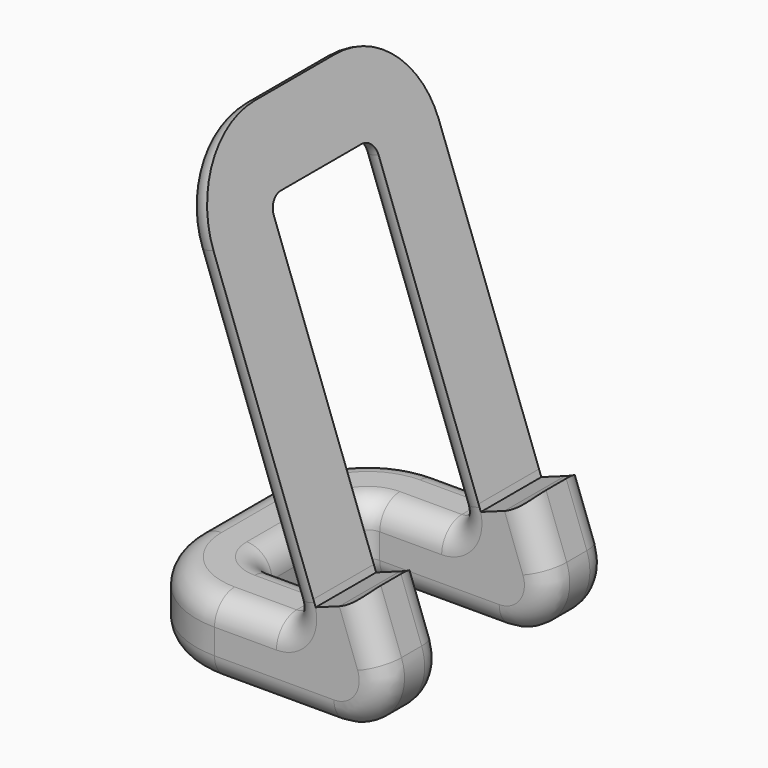
from build123d import *

# Parameters (mm, degrees)
F1_DEPTH     = 56
F2_W         = 41
F2_H         = 26
F3_DEPTH     = 15
F4_W         = 26
F4_H         = 80
F5_DEPTH     = 15
F6_R         = 10
F7_R         = 18
F8_R         = 3
F9_T1_DEPTH  = 58.556339633
F9_T3_DEPTH  = 12.2933358786
F9_T5_DEPTH  = 23.7185199326
F9_T7_DEPTH  = 24.4815236869
F9_T9_DEPTH  = 20
F9_T11_DEPTH = 58.556339633
F9_T13_DEPTH = 24.4815236869
F9_T16_ANGLE = 90
F9_T18_ANGLE = 110
F9_T20_ANGLE = 110
F9_T22_ANGLE = 110
F9_T24_ANGLE = 90
F9_T26_ANGLE = 90
F9_T28_ANGLE = 90
F9_T30_ANGLE = 90
F9_T32_ANGLE = 110
F9_T34_ANGLE = 90
F9_T36_ANGLE = 90
F9_T38_ANGLE = 90
F9_T40_ANGLE = 90
F9_T42_ANGLE = 90
F9_T44_ANGLE = 90
F9_T46_ANGLE = 90
F9_T48_ANGLE = 110
F9_T50_ANGLE = 110
F9_T52_ANGLE = 110
F9_T54_ANGLE = 110


# Not quite as in the source:
# - a fillet or chamfer that OpenCascade refuses, or shapes differently, is made with other operations: its cross-section is extruded or revolved along the edge and cut away or added


with BuildPart() as f1:
    # F0 (on Front) → F1 (new body)
    with BuildSketch(Plane.XZ):
        with BuildLine():
            Line((37.6205974839, 21.2589493944), (11.6270665912, 92.6755885741))
            Line((11.6270665912, 92.6755885741), (6.9286034872, 90.9654878575))
            Line((6.9286034872, 90.9654878575), (34.5777798989, 15))
            Line((34.5777798989, 15), (0, 15))
            Line((0, 15), (0, 0))
            Line((0, 0), (56, 0))
            Line((56, 0), (47.0175236918, 24.6791508276))
            ThreePointArc((47.0175236918, 24.6791508276), (45.0928436241, 22.9155064816), (42.7772806938, 21.7101007166))
            Line((42.7772806938, 21.7101007166), (38.0788175899, 20))
            Line((38.0788175899, 20), (37.6205974839, 21.2589493944))
        make_face()
    extrude(amount=F1_DEPTH)

    # F2 (on face) → F3 (cut, through all)
    with BuildSketch(Plane(origin=(0, 0, 0), x_dir=(1, 0, 0), z_dir=(0, 0, -1))):
        with Locations((35.5, 28)):
            Rectangle(F2_W, F2_H)
    extrude(amount=-F3_DEPTH, mode=Mode.SUBTRACT)

    # F4 (on face) → F5 (cut, through all)
    with BuildSketch(Plane(origin=(35.3538550955, 0, 12.8677509213), x_dir=(0, -1, 0), z_dir=(-0.9396926208, 0, -0.3420201433))):
        with Locations((28, 28.1098757281)):
            Rectangle(F4_W, F4_H)
    extrude(amount=-F5_DEPTH, mode=Mode.SUBTRACT)

    # F6
    f6_edges = [f1.edges().sort_by_distance(p)[0] for p in [
        (56, -7.5, 0),
        (56, -48.5, 0),
    ]]
    fillet(f6_edges, radius=F6_R)

    # F7
    f7_edges = [f1.edges().sort_by_distance(p)[0] for p in [
        (0, -56, 7.5),
        (0, 0, 7.5),
        (9.277835, -56, 91.820538),
        (9.277835, 0, 91.820538),
    ]]
    fillet(f7_edges, radius=F7_R)

    # F8
    f8_edges = [f1.edges().sort_by_distance(p)[0] for p in [
        (15, -15, 7.5),
        (15, -41, 7.5),
        (14.408137, -15, 77.725149),
        (14.408137, -41, 77.725149),
        (34.57778, -7.5, 15),
        (34.57778, -48.5, 15),
    ]]
    fillet(f8_edges, radius=F8_R)

    # F9: fillet of radius 5 on 42 edges, made by hand

    # F9_s2 → F9_t1 (cut)
    with BuildSketch(Plane(origin=(-22.2688890284, 0, 61.183269762), x_dir=(0, 1, 0), z_dir=(0.3420201433, 0, -0.9396926208))):
        with BuildLine():
            ThreePointArc((-51, 37.622786764), (-54.5355339059, 39.0872528581), (-56, 42.622786764))
            Line((-56, 42.622786764), (-56, 37.622786764))
            Line((-56, 37.622786764), (-51, 37.622786764))
        make_face()
        with BuildLine():
            ThreePointArc((0, 42.622786764), (-1.4644660941, 39.0872528581), (-5, 37.622786764))
            Line((-5, 37.622786764), (0, 37.622786764))
            Line((0, 37.622786764), (0, 42.622786764))
        make_face()
        with BuildLine():
            ThreePointArc((-10, 37.622786764), (-13.5355339059, 39.0872528581), (-15, 42.622786764))
            Line((-15, 42.622786764), (-15, 37.622786764))
            Line((-15, 37.622786764), (-10, 37.622786764))
        make_face()
    extrude(amount=F9_T1_DEPTH, mode=Mode.SUBTRACT)

    # F9_s4 → F9_t3 (cut)
    with BuildSketch(Plane.YZ.offset(18)):
        with BuildLine():
            ThreePointArc((-10, 15), (-13.5355339059, 13.5355339059), (-15, 10))
            Line((-15, 10), (-15, 15))
            Line((-15, 15), (-10, 15))
        make_face()
        with BuildLine():
            ThreePointArc((0, 10), (-1.4644660941, 13.5355339059), (-5, 15))
            Line((-5, 15), (0, 15))
            Line((0, 15), (0, 10))
        make_face()
        with BuildLine():
            ThreePointArc((-51, 15), (-54.5355339059, 13.5355339059), (-56, 10))
            Line((-56, 10), (-56, 15))
            Line((-56, 15), (-51, 15))
        make_face()
        with BuildLine():
            ThreePointArc((-46, 15), (-42.4644660941, 13.5355339059), (-41, 10))
            Line((-41, 10), (-41, 15))
            Line((-41, 15), (-46, 15))
        make_face()
    extrude(amount=F9_T3_DEPTH, mode=Mode.SUBTRACT)

    # F9_s6 → F9_t5 (cut)
    with BuildSketch(Plane.YZ.offset(18)):
        with BuildLine():
            ThreePointArc((0, 5), (-1.4644660941, 1.4644660941), (-5, 0))
            Line((-5, 0), (0, 0))
            Line((0, 0), (0, 5))
        make_face()
        with BuildLine():
            ThreePointArc((-10, 0), (-13.5355339059, 1.4644660941), (-15, 5))
            Line((-15, 5), (-15, 0))
            Line((-15, 0), (-10, 0))
        make_face()
        with BuildLine():
            ThreePointArc((-46, 0), (-42.4644660941, 1.4644660941), (-41, 5))
            Line((-41, 5), (-41, 0))
            Line((-41, 0), (-46, 0))
        make_face()
        with BuildLine():
            ThreePointArc((-51, 0), (-54.5355339059, 1.4644660941), (-56, 5))
            Line((-56, 5), (-56, 0))
            Line((-56, 0), (-51, 0))
        make_face()
    extrude(amount=F9_T5_DEPTH, mode=Mode.SUBTRACT)

    # F9_s8 → F9_t7 (cut)
    with BuildSketch(Plane(origin=(1.6662017331, 0, -4.577851638), x_dir=(0, 1, 0), z_dir=(-0.3420201433, 0, 0.9396926208))):
        with BuildLine():
            ThreePointArc((0, -47.622786764), (-1.4644660941, -51.1583206699), (-5, -52.622786764))
            Line((-5, -52.622786764), (0, -52.622786764))
            Line((0, -52.622786764), (0, -47.622786764))
        make_face()
        with BuildLine():
            ThreePointArc((-10, -52.622786764), (-13.5355339059, -51.1583206699), (-15, -47.622786764))
            Line((-15, -47.622786764), (-15, -52.622786764))
            Line((-15, -52.622786764), (-10, -52.622786764))
        make_face()
        with BuildLine():
            ThreePointArc((-56, -47.622786764), (-54.5355339059, -51.1583206699), (-51, -52.622786764))
            Line((-51, -52.622786764), (-56, -52.622786764))
            Line((-56, -52.622786764), (-56, -47.622786764))
        make_face()
    extrude(amount=F9_T7_DEPTH, mode=Mode.SUBTRACT)

    # F9_s10 → F9_t9 (cut)
    with BuildSketch(Plane.XZ.offset(18)):
        with BuildLine():
            ThreePointArc((5, 15), (1.4644660941, 13.5355339059), (0, 10))
            Line((0, 10), (0, 15))
            Line((0, 15), (5, 15))
        make_face()
        with BuildLine():
            ThreePointArc((10, 15), (13.5355339059, 13.5355339059), (15, 10))
            Line((15, 10), (15, 15))
            Line((15, 15), (10, 15))
        make_face()
        with BuildLine():
            ThreePointArc((8.6387042039, 86.2670247535), (8.8056283726, 90.0902167789), (11.6270665912, 92.6755885741))
            Line((11.6270665912, 92.6755885741), (6.9286034872, 90.9654878575))
            Line((6.9286034872, 90.9654878575), (8.6387042039, 86.2670247535))
        make_face()
        with BuildLine():
            ThreePointArc((10.3488049205, 81.5685616496), (12.9341767157, 78.7471234311), (16.7573687411, 78.5801992623))
            Line((16.7573687411, 78.5801992623), (12.0589056371, 76.8700985457))
            Line((12.0589056371, 76.8700985457), (10.3488049205, 81.5685616496))
        make_face()
        with BuildLine():
            ThreePointArc((10, 0), (13.5355339059, 1.4644660941), (15, 5))
            Line((15, 5), (15, 0))
            Line((15, 0), (10, 0))
        make_face()
        with BuildLine():
            ThreePointArc((5, 0), (1.4644660941, 1.4644660941), (0, 5))
            Line((0, 5), (0, 0))
            Line((0, 0), (5, 0))
        make_face()
    extrude(amount=F9_T9_DEPTH, mode=Mode.SUBTRACT)

    # F9_s12 → F9_t11 (cut)
    with BuildSketch(Plane(origin=(-2.2414413545, 0, 6.1583095086), x_dir=(0, 1, 0), z_dir=(-0.3420201433, 0, 0.9396926208))):
        with BuildLine():
            ThreePointArc((-46, -37.622786764), (-42.4644660941, -39.0872528581), (-41, -42.622786764))
            Line((-41, -42.622786764), (-41, -37.622786764))
            Line((-41, -37.622786764), (-46, -37.622786764))
        make_face()
    extrude(amount=F9_T11_DEPTH, mode=Mode.SUBTRACT)

    # F9_s14 → F9_t13 (cut)
    with BuildSketch(Plane(origin=(-6.7069725071, 0, 18.4272555162), x_dir=(0, 1, 0), z_dir=(0.3420201433, 0, -0.9396926208))):
        with BuildLine():
            ThreePointArc((-41, 47.622786764), (-42.4644660941, 51.1583206699), (-46, 52.622786764))
            Line((-46, 52.622786764), (-41, 52.622786764))
            Line((-41, 52.622786764), (-41, 47.622786764))
        make_face()
    extrude(amount=F9_T13_DEPTH, mode=Mode.SUBTRACT)

    # F9_s15 → F9_t16 (revolve, cut)
    with BuildSketch(Plane.XZ.offset(38)):
        with BuildLine():
            ThreePointArc((5, 0), (1.4644660941, 1.4644660941), (0, 5))
            Line((0, 5), (0, 0))
            Line((0, 0), (5, 0))
        make_face()
    revolve(axis=Axis((18, -38, 0), (0, 0, 1)), revolution_arc=F9_T16_ANGLE, mode=Mode.SUBTRACT)

    # F9_s17 → F9_t18 (revolve, cut)
    with BuildSketch(Plane(origin=(1.6662017331, 0, -4.577851638), x_dir=(0, 1, 0), z_dir=(-0.3420201433, 0, 0.9396926208))):
        with BuildLine():
            ThreePointArc((-10, -52.622786764), (-13.5355339059, -51.1583206699), (-15, -47.622786764))
            Line((-15, -47.622786764), (-15, -52.622786764))
            Line((-15, -52.622786764), (-10, -52.622786764))
        make_face()
    revolve(axis=Axis((41.7185199326, -15, 10), (0, 1, 0)), revolution_arc=F9_T18_ANGLE, mode=Mode.SUBTRACT)

    # F9_s19 → F9_t20 (revolve, cut)
    with BuildSketch(Plane.YZ.offset(30.2933358786)):
        with BuildLine():
            ThreePointArc((0, 10), (-1.4644660941, 13.5355339059), (-5, 15))
            Line((-5, 15), (0, 15))
            Line((0, 15), (0, 10))
        make_face()
    revolve(axis=Axis((30.2933358786, 0, 18), (0, -1, 0)), revolution_arc=F9_T20_ANGLE, mode=Mode.SUBTRACT)

    # F9_s21 → F9_t22 (revolve, cut)
    with BuildSketch(Plane(origin=(1.6662017331, 0, -4.577851638), x_dir=(0, 1, 0), z_dir=(-0.3420201433, 0, 0.9396926208))):
        with BuildLine():
            ThreePointArc((0, -47.622786764), (-1.4644660941, -51.1583206699), (-5, -52.622786764))
            Line((-5, -52.622786764), (0, -52.622786764))
            Line((0, -52.622786764), (0, -47.622786764))
        make_face()
    revolve(axis=Axis((41.7185199326, 0, 10), (0, 1, 0)), revolution_arc=F9_T22_ANGLE, mode=Mode.SUBTRACT)

    # F9_s23 → F9_t24 (revolve, cut)
    with BuildSketch(Plane.YZ.offset(18)):
        with BuildLine():
            ThreePointArc((-5, 15), (-1.4644660941, 13.5355339059), (0, 10))
            Line((0, 10), (0, 15))
            Line((0, 15), (-5, 15))
        make_face()
    revolve(axis=Axis((18, -18, 15), (0, 0, 1)), revolution_arc=F9_T24_ANGLE, mode=Mode.SUBTRACT)

    # F9_s25 → F9_t26 (revolve, cut)
    with BuildSketch(Plane.YZ.offset(18)):
        with BuildLine():
            ThreePointArc((-10, 15), (-13.5355339059, 13.5355339059), (-15, 10))
            Line((-15, 10), (-15, 15))
            Line((-15, 15), (-10, 15))
        make_face()
    revolve(axis=Axis((18, -18, 15), (0, 0, 1)), revolution_arc=F9_T26_ANGLE, mode=Mode.SUBTRACT)

    # F9_s27 → F9_t28 (revolve, cut)
    with BuildSketch(Plane.XZ.offset(38)):
        with BuildLine():
            ThreePointArc((5, 15), (1.4644660941, 13.5355339059), (0, 10))
            Line((0, 10), (0, 15))
            Line((0, 15), (5, 15))
        make_face()
    revolve(axis=Axis((18, -38, 15), (0, 0, 1)), revolution_arc=F9_T28_ANGLE, mode=Mode.SUBTRACT)

    # F9_s29 → F9_t30 (revolve, cut)
    with BuildSketch(Plane.XZ.offset(38)):
        with BuildLine():
            ThreePointArc((10, 15), (13.5355339059, 13.5355339059), (15, 10))
            Line((15, 10), (15, 15))
            Line((15, 15), (10, 15))
        make_face()
    revolve(axis=Axis((18, -38, 15), (0, 0, 1)), revolution_arc=F9_T30_ANGLE, mode=Mode.SUBTRACT)

    # F9_s31 → F9_t32 (revolve, cut)
    with BuildSketch(Plane.YZ.offset(30.2933358786)):
        with BuildLine():
            ThreePointArc((-10, 15), (-13.5355339059, 13.5355339059), (-15, 10))
            Line((-15, 10), (-15, 15))
            Line((-15, 15), (-10, 15))
        make_face()
    revolve(axis=Axis((30.2933358786, -15, 18), (0, -1, 0)), revolution_arc=F9_T32_ANGLE, mode=Mode.SUBTRACT)

    # F9_s33 → F9_t34 (revolve, cut)
    with BuildSketch(Plane.YZ.offset(18)):
        with BuildLine():
            ThreePointArc((0, 5), (-1.4644660941, 1.4644660941), (-5, 0))
            Line((-5, 0), (0, 0))
            Line((0, 0), (0, 5))
        make_face()
    revolve(axis=Axis((18, -18, 0), (0, 0, 1)), revolution_arc=F9_T34_ANGLE, mode=Mode.SUBTRACT)

    # F9_s35 → F9_t36 (revolve, cut)
    with BuildSketch(Plane(origin=(-22.2688890284, 0, 61.183269762), x_dir=(0, 1, 0), z_dir=(0.3420201433, 0, -0.9396926208))):
        with BuildLine():
            ThreePointArc((-5, 37.622786764), (-1.4644660941, 39.0872528581), (0, 42.622786764))
            Line((0, 42.622786764), (0, 37.622786764))
            Line((0, 37.622786764), (-5, 37.622786764))
        make_face()
    revolve(axis=Axis((13.0849660671, -18, 74.0510206833), (0.9396926208, 0, 0.3420201433)), revolution_arc=F9_T36_ANGLE, mode=Mode.SUBTRACT)

    # F9_s37 → F9_t38 (revolve, cut)
    with BuildSketch(Plane(origin=(-22.2688890284, 0, 61.183269762), x_dir=(0, 1, 0), z_dir=(0.3420201433, 0, -0.9396926208))):
        with BuildLine():
            ThreePointArc((-10, 37.622786764), (-13.5355339059, 39.0872528581), (-15, 42.622786764))
            Line((-15, 42.622786764), (-15, 37.622786764))
            Line((-15, 37.622786764), (-10, 37.622786764))
        make_face()
    revolve(axis=Axis((13.0849660671, -18, 74.0510206833), (0.9396926208, 0, 0.3420201433)), revolution_arc=F9_T38_ANGLE, mode=Mode.SUBTRACT)

    # F9_s39 → F9_t40 (revolve, cut)
    with BuildSketch(Plane.XZ.offset(38)):
        with BuildLine():
            ThreePointArc((8.6387042039, 86.2670247535), (8.8056283726, 90.0902167789), (11.6270665912, 92.6755885741))
            Line((11.6270665912, 92.6755885741), (6.9286034872, 90.9654878575))
            Line((6.9286034872, 90.9654878575), (8.6387042039, 86.2670247535))
        make_face()
    revolve(axis=Axis((13.0849660671, -38, 74.0510206833), (0.9396926208, 0, 0.3420201433)), revolution_arc=F9_T40_ANGLE, mode=Mode.SUBTRACT)

    # F9_s41 → F9_t42 (revolve, cut)
    with BuildSketch(Plane(origin=(-22.2688890284, 0, 61.183269762), x_dir=(0, 1, 0), z_dir=(0.3420201433, 0, -0.9396926208))):
        with BuildLine():
            ThreePointArc((-46, 37.622786764), (-42.4644660941, 39.0872528581), (-41, 42.622786764))
            Line((-41, 42.622786764), (-41, 37.622786764))
            Line((-41, 37.622786764), (-46, 37.622786764))
        make_face()
    revolve(axis=Axis((13.0849660671, -38, 74.0510206833), (-0.9396926208, 0, -0.3420201433)), revolution_arc=F9_T42_ANGLE, mode=Mode.SUBTRACT)

    # F9_s43 → F9_t44 (revolve, cut)
    with BuildSketch(Plane.YZ.offset(18)):
        with BuildLine():
            ThreePointArc((-10, 0), (-13.5355339059, 1.4644660941), (-15, 5))
            Line((-15, 5), (-15, 0))
            Line((-15, 0), (-10, 0))
        make_face()
    revolve(axis=Axis((18, -18, 0), (0, 0, 1)), revolution_arc=F9_T44_ANGLE, mode=Mode.SUBTRACT)

    # F9_s45 → F9_t46 (revolve, cut)
    with BuildSketch(Plane.XZ.offset(38)):
        with BuildLine():
            ThreePointArc((10, 0), (13.5355339059, 1.4644660941), (15, 5))
            Line((15, 5), (15, 0))
            Line((15, 0), (10, 0))
        make_face()
    revolve(axis=Axis((18, -38, 0), (0, 0, 1)), revolution_arc=F9_T46_ANGLE, mode=Mode.SUBTRACT)

    # F9_s47 → F9_t48 (revolve, cut)
    with BuildSketch(Plane.YZ.offset(30.2933358786)):
        with BuildLine():
            ThreePointArc((-56, 10), (-54.5355339059, 13.5355339059), (-51, 15))
            Line((-51, 15), (-56, 15))
            Line((-56, 15), (-56, 10))
        make_face()
    revolve(axis=Axis((30.2933358786, -56, 18), (0, -1, 0)), revolution_arc=F9_T48_ANGLE, mode=Mode.SUBTRACT)

    # F9_s49 → F9_t50 (revolve, cut)
    with BuildSketch(Plane.YZ.offset(41.7185199326)):
        with BuildLine():
            ThreePointArc((-56, 5), (-54.5355339059, 1.4644660941), (-51, 0))
            Line((-51, 0), (-56, 0))
            Line((-56, 0), (-56, 5))
        make_face()
    revolve(axis=Axis((41.7185199326, -56, 10), (0, -1, 0)), revolution_arc=F9_T50_ANGLE, mode=Mode.SUBTRACT)

    # F9_s51 → F9_t52 (revolve, cut)
    with BuildSketch(Plane.YZ.offset(30.2933358786)):
        with BuildLine():
            ThreePointArc((-46, 15), (-42.4644660941, 13.5355339059), (-41, 10))
            Line((-41, 10), (-41, 15))
            Line((-41, 15), (-46, 15))
        make_face()
    revolve(axis=Axis((30.2933358786, -41, 18), (0, -1, 0)), revolution_arc=F9_T52_ANGLE, mode=Mode.SUBTRACT)

    # F9_s53 → F9_t54 (revolve, cut)
    with BuildSketch(Plane.YZ.offset(41.7185199326)):
        with BuildLine():
            ThreePointArc((-41, 5), (-42.4644660941, 1.4644660941), (-46, 0))
            Line((-46, 0), (-41, 0))
            Line((-41, 0), (-41, 5))
        make_face()
    revolve(axis=Axis((41.7185199326, -41, 10), (0, -1, 0)), revolution_arc=F9_T54_ANGLE, mode=Mode.SUBTRACT)


solid = f1.part
